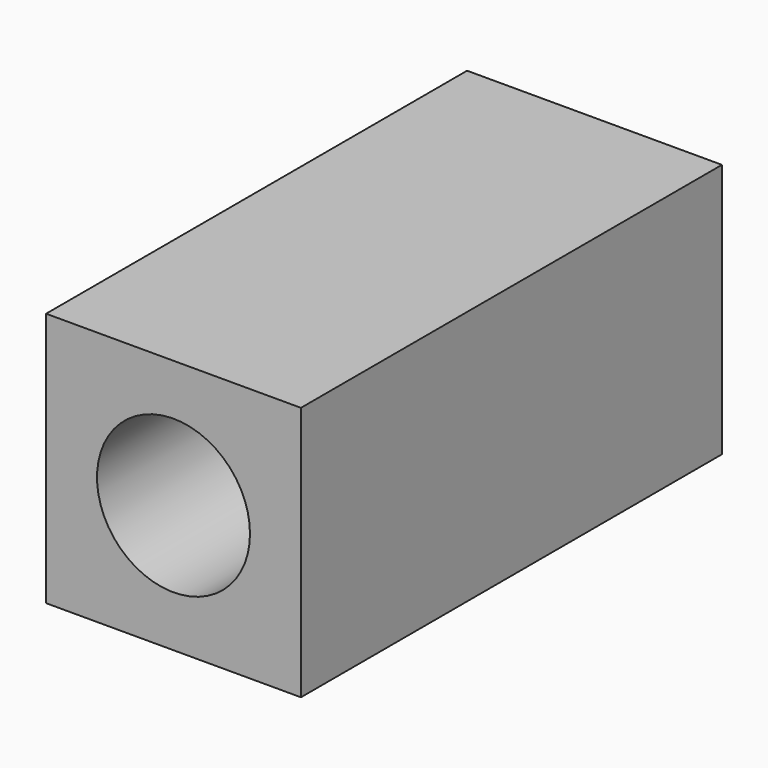
from build123d import *

# Parameters (mm, degrees)
F0_W     = 20
F0_H     = 20
F1_DEPTH = 41.3
F2_R     = 6.0024367581
F3_DEPTH = 41.301


# Not quite as in the source:
# - a feature of the source that left no trace in its solid (it failed there, or was rolled back) is left out


with BuildPart() as f1:
    # F0 (on Front) → F1 (new body)
    with BuildSketch(Plane.XZ):
        Rectangle(F0_W, F0_H)
    extrude(amount=F1_DEPTH)

    # F2 (on face) → F3 (cut, through all)
    with BuildSketch(Plane.XZ.offset(41.3)):
        Circle(F2_R)
    extrude(amount=-F3_DEPTH, mode=Mode.SUBTRACT)


solid = f1.part
